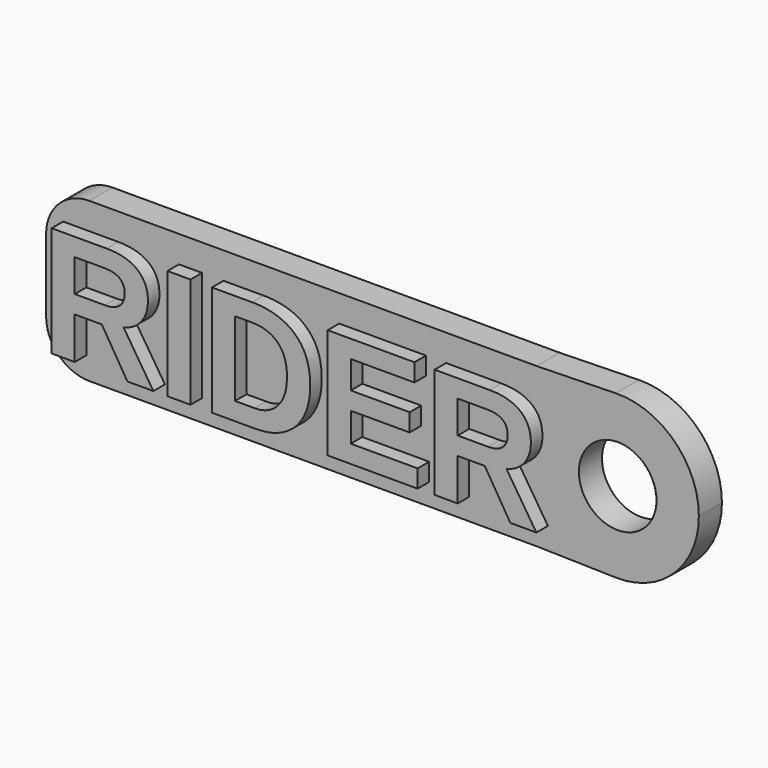
from build123d import *

# Parameters (mm, degrees)
F0_TEXT_SIZE = 11.1111111111
F1_DEPTH     = 1
F2_R         = 2.69
F3_DEPTH     = 2
F4_R         = 3


# Not quite as in the source:
# - Text() gives the source's letters only with a copy of the font that has no kerning and outlines rounded to 1/6400 em; it was checked with that copy


with BuildPart() as f1:
    # F0 (on Front) → F1 (new body)
    with BuildSketch(Plane.XZ):
        with Locations((-17.5572916667, -8)):
            Text('RIDER', F0_TEXT_SIZE, font='Arimo', font_style=FontStyle.BOLD, text_align=(TextAlign.LEFT, TextAlign.BOTTOM))
    extrude(amount=F1_DEPTH)


with BuildPart() as f3:
    # F2 (on Front) → F3 (new body)
    with BuildSketch(Plane.XZ):
        with BuildLine():
            Line((-18, -9.5), (16, -9.5))
            Line((16, -9.5), (21.4986114618, -9.6235799041))
            ThreePointArc((21.4986114618, -9.6235799041), (16, -4), (21.4986114618, 1.6235799041))
            Line((21.4986114618, 1.6235799041), (16, 1.5))
            Line((16, 1.5), (-18, 1.5))
            Line((-18, 1.5), (-18, -9.5))
        make_face()
        with BuildLine():
            ThreePointArc((21.4986114618, 1.6235799041), (16, -4), (21.4986114618, -9.6235799041))
            ThreePointArc((21.4986114618, -9.6235799041), (25.5575366796, -8.0219125132), (27.25, -4))
            ThreePointArc((27.25, -4), (25.5575366796, 0.0219125132), (21.4986114618, 1.6235799041))
        make_face()
        with Locations((21.625, -4)):
            Circle(F2_R, mode=Mode.SUBTRACT)
    extrude(amount=-F3_DEPTH)

    # F4
    f4_edges = [f3.edges().sort_by_distance(p)[0] for p in [
        (-18, 1, 1.5),
        (-18, 1, -9.5),
        (16, 1, -9.5),
        (16, 1, 1.5),
    ]]
    fillet(f4_edges, radius=F4_R)


solid = Compound([f1.part, f3.part])
